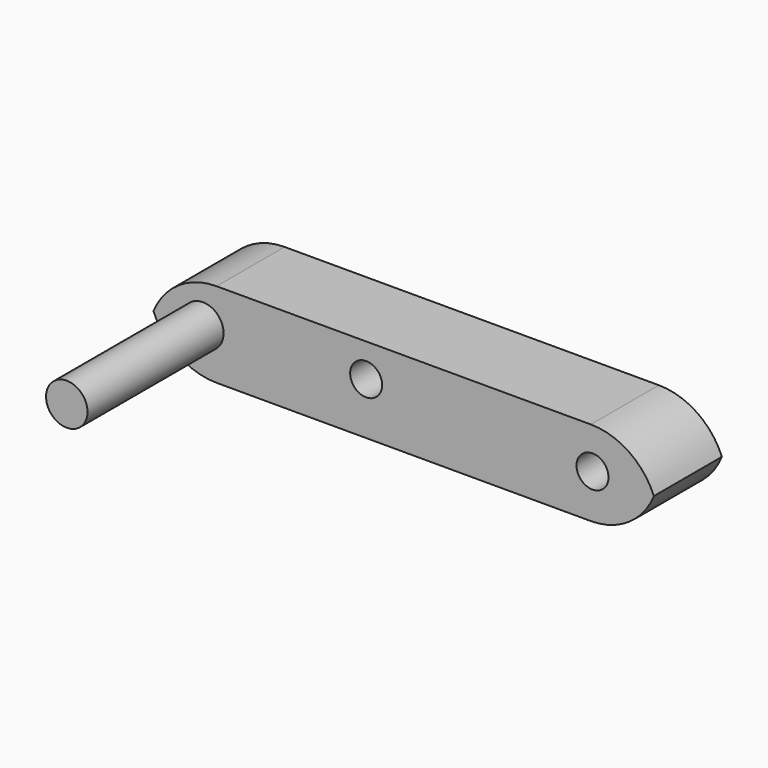
from build123d import *

# Parameters (mm, degrees)
F0_W        = 38.1
F0_H        = 6.35
F0_R        = 1.1938
F1_DEPTH    = 6.35
F2_T1_DEPTH = 31.75
F3_R        = 1.547841459
F4_DEPTH    = 12.7


# Not quite as in the source:
# - a fillet or chamfer that OpenCascade refuses, or shapes differently, is made with other operations: its cross-section is extruded or revolved along the edge and cut away or added


with BuildPart() as f1:
    # F0 (on Front) → F1 (new body)
    with BuildSketch(Plane.XZ):
        with Locations((19.05, 3.175)):
            Rectangle(F0_W, F0_H)
        with Locations((16.2474811077, 3.8697349373)):
            Circle(F0_R, mode=Mode.SUBTRACT)
        with Locations((33.1476069987, 3.302)):
            Circle(F0_R, mode=Mode.SUBTRACT)
    extrude(amount=F1_DEPTH)

    # F2: fillet of radius 5.08 on 4 edges, made by hand

    # F2_s2 → F2_t1 (cut)
    with BuildSketch(Plane.XZ.offset(-12.7)):
        with BuildLine():
            ThreePointArc((0, 1.27), (1.4878975516, 4.8621024484), (5.08, 6.35))
            Line((5.08, 6.35), (0, 6.35))
            Line((0, 6.35), (0, 1.27))
        make_face()
        with BuildLine():
            ThreePointArc((0, 5.08), (1.4878975516, 1.4878975516), (5.08, 0))
            Line((5.08, 0), (0, 0))
            Line((0, 0), (0, 5.08))
        make_face()
        with BuildLine():
            ThreePointArc((38.1, 1.27), (36.6121024484, 4.8621024484), (33.02, 6.35))
            Line((33.02, 6.35), (38.1, 6.35))
            Line((38.1, 6.35), (38.1, 1.27))
        make_face()
        with BuildLine():
            ThreePointArc((33.02, 0), (36.6121024484, 1.4878975516), (38.1, 5.08))
            Line((38.1, 5.08), (38.1, 0))
            Line((38.1, 0), (33.02, 0))
        make_face()
    extrude(amount=F2_T1_DEPTH, mode=Mode.SUBTRACT)

    # F3 (on face) → F4 (join)
    with BuildSketch(Plane.XZ.offset(6.35)):
        with Locations((4.0558986366, 3.4221061505)):
            Circle(F3_R)
    extrude(amount=F4_DEPTH)


solid = f1.part
